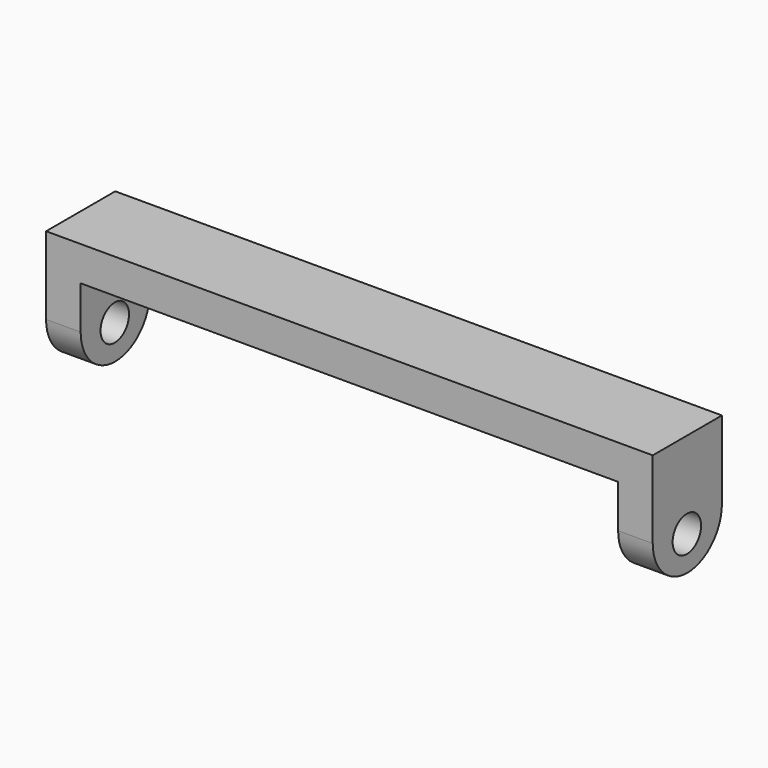
from build123d import *

# Parameters (mm, degrees)
F0_W        = 49.2125
F0_H        = 7.9375
F1_DEPTH    = 3.175
F2_DEPTH    = 3.302
F3_DEPTH    = 3.175
F4_W        = 3.175
F4_H        = 7.9375
F5_DEPTH    = 7.9375
F7_D        = 3.2639
F8_T1_DEPTH = 23.114
F8_T3_DEPTH = 23.114


# Not quite as in the source:
# - a fillet or chamfer that OpenCascade refuses, or shapes differently, is made with other operations: its cross-section is extruded or revolved along the edge and cut away or added


with BuildPart() as f1:
    # F0 (on Top) → F1 (new body)
    with BuildSketch(Plane.XY):
        with Locations((-5.1108673215, 16.8213252627)):
            Rectangle(F0_W, F0_H)
    extrude(amount=F1_DEPTH)

    # F2 (add): a face of the model
    f2_faces = [f1.faces().sort_by_distance(p)[0] for p in [
        (19.4953826785, 16.8213252627, 1.5875),
    ]]
    extrude(f2_faces, amount=F2_DEPTH)

    # F3 (add): a face of the model
    f3_faces = [f1.faces().sort_by_distance(p)[0] for p in [
        (-29.7171173215, 16.8213252627, 1.5875),
    ]]
    extrude(f3_faces, amount=F3_DEPTH)

    # F4 (on face) → F5 (join)
    with BuildSketch(Plane(origin=(0, 0, 0), x_dir=(1, 0, 0), z_dir=(0, 0, -1))):
        with Locations((21.2098826785, -16.8213252627)):
            Rectangle(F4_W, F4_H)
        with Locations((-31.3046173215, -16.8213252627)):
            Rectangle(F4_W, F4_H)
    extrude(amount=F5_DEPTH)

    # F7 (through all)
    with Locations(Plane.YZ.offset(22.7973826785)):
        with Locations((16.7667926535, -4.7623126715)):
            Hole(F7_D / 2)

    # F8: fillet of radius 3.9878 on 4 edges, made by hand

    # F8_s2 → F8_t1 (cut)
    with BuildSketch(Plane.YZ.offset(9.6528826785)):
        with BuildLine():
            ThreePointArc((12.8525752627, -3.9497), (14.0205748406, -6.769500422), (16.8403752627, -7.9375))
            Line((16.8403752627, -7.9375), (12.8525752627, -7.9375))
            Line((12.8525752627, -7.9375), (12.8525752627, -3.9497))
        make_face()
        with BuildLine():
            ThreePointArc((20.7900752627, -3.9497), (19.6220756847, -6.769500422), (16.8022752627, -7.9375))
            Line((16.8022752627, -7.9375), (20.7900752627, -7.9375))
            Line((20.7900752627, -7.9375), (20.7900752627, -3.9497))
        make_face()
    extrude(amount=F8_T1_DEPTH, mode=Mode.SUBTRACT)

    # F8_s4 → F8_t3 (cut)
    with BuildSketch(Plane.YZ.offset(-42.8616173215)):
        with BuildLine():
            ThreePointArc((12.8525752627, -3.9497), (14.0205748406, -6.769500422), (16.8403752627, -7.9375))
            Line((16.8403752627, -7.9375), (12.8525752627, -7.9375))
            Line((12.8525752627, -7.9375), (12.8525752627, -3.9497))
        make_face()
        with BuildLine():
            ThreePointArc((20.7900752627, -3.9497), (19.6220756847, -6.769500422), (16.8022752627, -7.9375))
            Line((16.8022752627, -7.9375), (20.7900752627, -7.9375))
            Line((20.7900752627, -7.9375), (20.7900752627, -3.9497))
        make_face()
    extrude(amount=F8_T3_DEPTH, mode=Mode.SUBTRACT)


solid = f1.part
